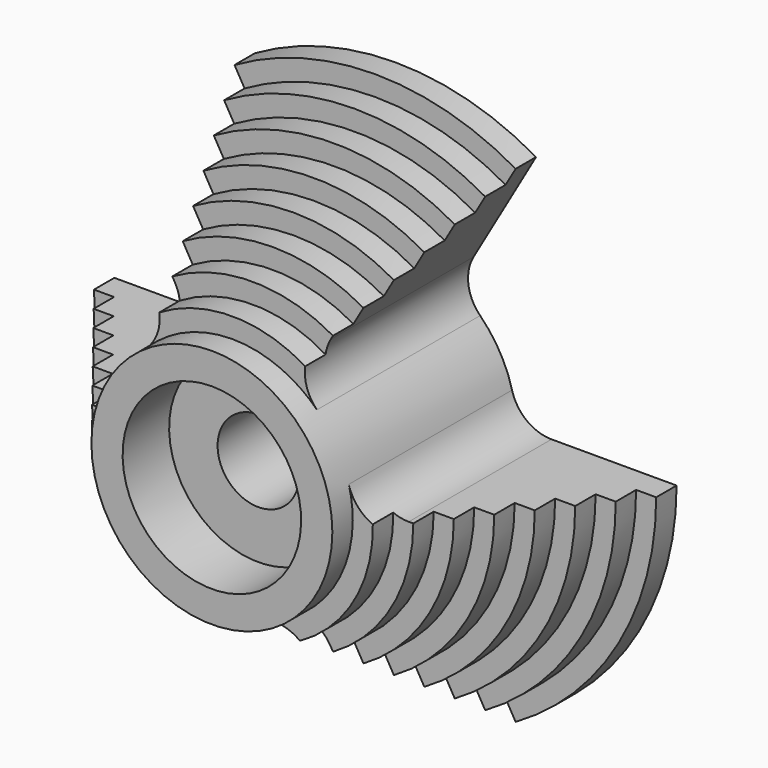
from build123d import *

# Parameters (mm, degrees)
F3_DEPTH      = 28.576
F4_T4_DEPTH   = 25.4
F4_S5_R       = 17.5
F4_T6_DEPTH   = 15
F4_T11_DEPTH  = 25.4
F4_S12_R      = 17.5
F4_T13_DEPTH  = 15
F4_T18_DEPTH  = 25.4
F4_S19_R      = 17.5
F4_T20_DEPTH  = 15
F4_T25_DEPTH  = 25.4
F4_S27_R      = 17.5
F4_T28_DEPTH  = 15
F4_T32_DEPTH  = 25.4
F4_S34_R      = 17.5
F4_T35_DEPTH  = 15
F4_T39_DEPTH  = 25.4
F4_S41_R      = 17.5
F4_T42_DEPTH  = 15
F4_T46_DEPTH  = 25.4
F4_S47_R      = 17.5
F4_T48_DEPTH  = 15
F4_T53_DEPTH  = 25.4
F4_S54_R      = 17.5
F4_T55_DEPTH  = 15
F4_T60_DEPTH  = 25.4
F4_S61_R      = 17.5
F4_T62_DEPTH  = 15
F4_T67_DEPTH  = 25.4
F4_S69_R      = 17.5
F4_T70_DEPTH  = 15
F4_T74_DEPTH  = 25.4
F4_S76_R      = 17.5
F4_T77_DEPTH  = 15
F4_T81_DEPTH  = 25.4
F4_S83_R      = 17.5
F4_T84_DEPTH  = 15
F4_T88_DEPTH  = 25.4
F4_S89_R      = 17.5
F4_T90_DEPTH  = 15
F4_T95_DEPTH  = 25.4
F4_S96_R      = 17.5
F4_T97_DEPTH  = 15
F4_T102_DEPTH = 25.4
F4_S103_R     = 17.5
F4_T104_DEPTH = 15
F4_T109_DEPTH = 25.4
F4_S111_R     = 17.5
F4_T112_DEPTH = 15
F4_T116_DEPTH = 25.4
F4_S118_R     = 17.5
F4_T119_DEPTH = 15
F4_T123_DEPTH = 25.4
F4_S125_R     = 17.5
F4_T126_DEPTH = 15


# Not quite as in the source:
# - a fillet or chamfer that OpenCascade refuses, or shapes differently, is made with other operations: its cross-section is extruded or revolved along the edge and cut away or added


with BuildPart() as f1:
    # F0 (on Right) → F1 (revolve)
    with BuildSketch(Plane.YZ):
        Polygon((0, 15), (0, 11.1125), (7.239, 11.1125), (7.239, 5.08), (21.336, 5.08), (21.336, 11.1125), (28.575, 11.1125), (28.575, 35), (25.4, 35), (25.4, 32.5), (22.225, 32.5), (22.225, 30), (19.05, 30), (19.05, 27.5), (15.875, 27.5), (15.875, 25), (12.7, 25), (12.7, 22.5), (9.525, 22.5), (9.525, 20), (6.35, 20), (6.35, 17.5), (3.175, 17.5), (3.175, 15), align=None)
    revolve(axis=Axis((0, 14.2875, 0), (0, 1, 0)))

    # F2 (on Front) → F3 (cut, through all)
    with BuildSketch(Plane.XZ):
        with BuildLine():
            ThreePointArc((-15, 0), (-12.9903810568, 7.5), (-7.5, 12.9903810568))
            Line((-7.5, 12.9903810568), (-17.5, 30.3108891325))
            ThreePointArc((-17.5, 30.3108891325), (-30.3108891325, 17.5), (-35, 0))
            Line((-35, 0), (-15, 0))
        make_face()
        with BuildLine():
            ThreePointArc((7.5, 12.9903810568), (12.9903810568, 7.5), (15, 0))
            Line((15, 0), (35, 0))
            ThreePointArc((35, 0), (30.3108891325, 17.5), (17.5, 30.3108891325))
            Line((17.5, 30.3108891325), (7.5, 12.9903810568))
        make_face()
        with BuildLine():
            Line((17.5, -30.3108891325), (7.5, -12.9903810568))
            ThreePointArc((7.5, -12.9903810568), (0, -15), (-7.5, -12.9903810568))
            Line((-7.5, -12.9903810568), (-17.5, -30.3108891325))
            ThreePointArc((-17.5, -30.3108891325), (0, -35), (17.5, -30.3108891325))
        make_face()
    extrude(amount=-F3_DEPTH, mode=Mode.SUBTRACT)

    # F4: fillet of radius 5.08 on 6 edges, made by hand


with BuildPart() as f4_tool2:
    # F4_s3 → F4_t4 (new body)
    with BuildSketch(Plane.XZ.offset(-3.175)):
        with BuildLine():
            ThreePointArc((19.4267856322, 0), (16.3221367597, 1.059110126), (14.5120410599, 3.7948207171))
            ThreePointArc((14.5120410599, 3.7948207171), (14.8775101394, 1.9130321614), (15, 0))
            Line((15, 0), (19.4267856322, 0))
        make_face()
    extrude(amount=-F4_T4_DEPTH)

    # F4_s5 → F4_t6 (intersect, symmetric)
    with BuildSketch(Plane.XZ.offset(-15.9)):
        Circle(F4_S5_R)
    extrude(amount=F4_T6_DEPTH, both=True, mode=Mode.INTERSECT)

    split(bisect_by=Plane.XZ.offset(-6.35), keep=Keep.TOP)


with BuildPart() as f1_1:
    add(f1.part)

    # F4_t1: union F4_tool2
    add(f4_tool2.part)


with BuildPart() as f4_tool9:
    # F4_s10 → F4_t11 (new body)
    with BuildSketch(Plane.XZ.offset(-3.175)):
        with BuildLine():
            ThreePointArc((19.4267856322, 0), (16.3221367597, 1.059110126), (14.5120410599, 3.7948207171))
            ThreePointArc((14.5120410599, 3.7948207171), (14.8775101394, 1.9130321614), (15, 0))
            Line((15, 0), (19.4267856322, 0))
        make_face()
    extrude(amount=-F4_T11_DEPTH)

    # F4_s12 → F4_t13 (cut, symmetric)
    with BuildSketch(Plane.XZ.offset(-15.9)):
        Circle(F4_S12_R)
    extrude(amount=F4_T13_DEPTH, both=True, mode=Mode.SUBTRACT)

    split(bisect_by=Plane.XZ.offset(-6.35), keep=Keep.BOTTOM)


with BuildPart() as f1_2:
    add(f1_1.part)

    # F4_t8: union F4_tool9
    add(f4_tool9.part)


with BuildPart() as f4_tool16:
    # F4_s17 → F4_t18 (new body)
    with BuildSketch(Plane.XZ.offset(-3.175)):
        with BuildLine():
            ThreePointArc((19.4267856322, 0), (16.3221367597, 1.059110126), (14.5120410599, 3.7948207171))
            ThreePointArc((14.5120410599, 3.7948207171), (14.8775101394, 1.9130321614), (15, 0))
            Line((15, 0), (19.4267856322, 0))
        make_face()
    extrude(amount=-F4_T18_DEPTH)

    # F4_s19 → F4_t20 (intersect, symmetric)
    with BuildSketch(Plane.XZ.offset(-15.9)):
        Circle(F4_S19_R)
    extrude(amount=F4_T20_DEPTH, both=True, mode=Mode.INTERSECT)

    split(bisect_by=Plane.XZ.offset(-6.35), keep=Keep.BOTTOM)


with BuildPart() as f1_3:
    add(f1_2.part)

    # F4_t15: union F4_tool16
    add(f4_tool16.part)


with BuildPart() as f4_tool23:
    # F4_s24 → F4_t25 (new body)
    with BuildSketch(Plane.XZ.offset(-3.175)):
        with BuildLine():
            ThreePointArc((9.7133928161, 16.8240898714), (9.0782846544, 13.6058300149), (10.5424316738, 10.6703858601))
            ThreePointArc((10.5424316738, 10.6703858601), (9.0954895198, 11.9277856451), (7.5, 12.9903810568))
            Line((7.5, 12.9903810568), (9.7133928161, 16.8240898714))
        make_face()
    extrude(amount=-F4_T25_DEPTH)

    split(bisect_by=Plane.XZ.offset(-6.35), keep=Keep.TOP)

    # F4_s27 → F4_t28 (intersect, symmetric)
    with BuildSketch(Plane.XZ.offset(-15.9)):
        Circle(F4_S27_R)
    extrude(amount=F4_T28_DEPTH, both=True, mode=Mode.INTERSECT)


with BuildPart() as f1_4:
    add(f1_3.part)

    # F4_t22: union F4_tool23
    add(f4_tool23.part)


with BuildPart() as f4_tool30:
    # F4_s31 → F4_t32 (new body)
    with BuildSketch(Plane.XZ.offset(-3.175)):
        with BuildLine():
            ThreePointArc((9.7133928161, 16.8240898714), (9.0782846544, 13.6058300149), (10.5424316738, 10.6703858601))
            ThreePointArc((10.5424316738, 10.6703858601), (9.0954895198, 11.9277856451), (7.5, 12.9903810568))
            Line((7.5, 12.9903810568), (9.7133928161, 16.8240898714))
        make_face()
    extrude(amount=-F4_T32_DEPTH)

    split(bisect_by=Plane.XZ.offset(-6.35), keep=Keep.BOTTOM)

    # F4_s34 → F4_t35 (cut, symmetric)
    with BuildSketch(Plane.XZ.offset(-15.9)):
        Circle(F4_S34_R)
    extrude(amount=F4_T35_DEPTH, both=True, mode=Mode.SUBTRACT)


with BuildPart() as f1_5:
    add(f1_4.part)

    # F4_t29: union F4_tool30
    add(f4_tool30.part)


with BuildPart() as f4_tool37:
    # F4_s38 → F4_t39 (new body)
    with BuildSketch(Plane.XZ.offset(-3.175)):
        with BuildLine():
            ThreePointArc((9.7133928161, 16.8240898714), (9.0782846544, 13.6058300149), (10.5424316738, 10.6703858601))
            ThreePointArc((10.5424316738, 10.6703858601), (9.0954895198, 11.9277856451), (7.5, 12.9903810568))
            Line((7.5, 12.9903810568), (9.7133928161, 16.8240898714))
        make_face()
    extrude(amount=-F4_T39_DEPTH)

    split(bisect_by=Plane.XZ.offset(-6.35), keep=Keep.BOTTOM)

    # F4_s41 → F4_t42 (intersect, symmetric)
    with BuildSketch(Plane.XZ.offset(-15.9)):
        Circle(F4_S41_R)
    extrude(amount=F4_T42_DEPTH, both=True, mode=Mode.INTERSECT)


with BuildPart() as f1_6:
    add(f1_5.part)

    # F4_t36: union F4_tool37
    add(f4_tool37.part)


with BuildPart() as f4_tool44:
    # F4_s45 → F4_t46 (new body)
    with BuildSketch(Plane.XZ.offset(-3.175)):
        with BuildLine():
            ThreePointArc((-10.5424316738, 10.6703858601), (-9.0782846544, 13.6058300149), (-9.7133928161, 16.8240898714))
            Line((-9.7133928161, 16.8240898714), (-7.5, 12.9903810568))
            ThreePointArc((-7.5, 12.9903810568), (-9.0954895198, 11.9277856451), (-10.5424316738, 10.6703858601))
        make_face()
    extrude(amount=-F4_T46_DEPTH)

    # F4_s47 → F4_t48 (intersect, symmetric)
    with BuildSketch(Plane.XZ.offset(-15.9)):
        Circle(F4_S47_R)
    extrude(amount=F4_T48_DEPTH, both=True, mode=Mode.INTERSECT)

    split(bisect_by=Plane.XZ.offset(-6.35), keep=Keep.TOP)


with BuildPart() as f1_7:
    add(f1_6.part)

    # F4_t43: union F4_tool44
    add(f4_tool44.part)


with BuildPart() as f4_tool51:
    # F4_s52 → F4_t53 (new body)
    with BuildSketch(Plane.XZ.offset(-3.175)):
        with BuildLine():
            ThreePointArc((-10.5424316738, 10.6703858601), (-9.0782846544, 13.6058300149), (-9.7133928161, 16.8240898714))
            Line((-9.7133928161, 16.8240898714), (-7.5, 12.9903810568))
            ThreePointArc((-7.5, 12.9903810568), (-9.0954895198, 11.9277856451), (-10.5424316738, 10.6703858601))
        make_face()
    extrude(amount=-F4_T53_DEPTH)

    # F4_s54 → F4_t55 (intersect, symmetric)
    with BuildSketch(Plane.XZ.offset(-15.9)):
        Circle(F4_S54_R)
    extrude(amount=F4_T55_DEPTH, both=True, mode=Mode.INTERSECT)

    split(bisect_by=Plane.XZ.offset(-6.35), keep=Keep.BOTTOM)


with BuildPart() as f1_8:
    add(f1_7.part)

    # F4_t50: union F4_tool51
    add(f4_tool51.part)


with BuildPart() as f4_tool58:
    # F4_s59 → F4_t60 (new body)
    with BuildSketch(Plane.XZ.offset(-3.175)):
        with BuildLine():
            ThreePointArc((-10.5424316738, 10.6703858601), (-9.0782846544, 13.6058300149), (-9.7133928161, 16.8240898714))
            Line((-9.7133928161, 16.8240898714), (-7.5, 12.9903810568))
            ThreePointArc((-7.5, 12.9903810568), (-9.0954895198, 11.9277856451), (-10.5424316738, 10.6703858601))
        make_face()
    extrude(amount=-F4_T60_DEPTH)

    # F4_s61 → F4_t62 (cut, symmetric)
    with BuildSketch(Plane.XZ.offset(-15.9)):
        Circle(F4_S61_R)
    extrude(amount=F4_T62_DEPTH, both=True, mode=Mode.SUBTRACT)

    split(bisect_by=Plane.XZ.offset(-6.35), keep=Keep.BOTTOM)


with BuildPart() as f1_9:
    add(f1_8.part)

    # F4_t57: union F4_tool58
    add(f4_tool58.part)


with BuildPart() as f4_tool65:
    # F4_s66 → F4_t67 (new body)
    with BuildSketch(Plane.XZ.offset(-3.175)):
        with BuildLine():
            ThreePointArc((-19.4267856322, 0), (-16.3221367597, 1.059110126), (-14.5120410599, 3.7948207171))
            ThreePointArc((-14.5120410599, 3.7948207171), (-14.8775101394, 1.9130321614), (-15, 0))
            Line((-15, 0), (-19.4267856322, 0))
        make_face()
    extrude(amount=-F4_T67_DEPTH)

    split(bisect_by=Plane.XZ.offset(-6.35), keep=Keep.TOP)

    # F4_s69 → F4_t70 (intersect, symmetric)
    with BuildSketch(Plane.XZ.offset(-15.9)):
        Circle(F4_S69_R)
    extrude(amount=F4_T70_DEPTH, both=True, mode=Mode.INTERSECT)


with BuildPart() as f1_10:
    add(f1_9.part)

    # F4_t64: union F4_tool65
    add(f4_tool65.part)


with BuildPart() as f4_tool72:
    # F4_s73 → F4_t74 (new body)
    with BuildSketch(Plane.XZ.offset(-3.175)):
        with BuildLine():
            ThreePointArc((-19.4267856322, 0), (-16.3221367597, 1.059110126), (-14.5120410599, 3.7948207171))
            ThreePointArc((-14.5120410599, 3.7948207171), (-14.8775101394, 1.9130321614), (-15, 0))
            Line((-15, 0), (-19.4267856322, 0))
        make_face()
    extrude(amount=-F4_T74_DEPTH)

    split(bisect_by=Plane.XZ.offset(-6.35), keep=Keep.BOTTOM)

    # F4_s76 → F4_t77 (cut, symmetric)
    with BuildSketch(Plane.XZ.offset(-15.9)):
        Circle(F4_S76_R)
    extrude(amount=F4_T77_DEPTH, both=True, mode=Mode.SUBTRACT)


with BuildPart() as f1_11:
    add(f1_10.part)

    # F4_t71: union F4_tool72
    add(f4_tool72.part)


with BuildPart() as f4_tool79:
    # F4_s80 → F4_t81 (new body)
    with BuildSketch(Plane.XZ.offset(-3.175)):
        with BuildLine():
            ThreePointArc((-19.4267856322, 0), (-16.3221367597, 1.059110126), (-14.5120410599, 3.7948207171))
            ThreePointArc((-14.5120410599, 3.7948207171), (-14.8775101394, 1.9130321614), (-15, 0))
            Line((-15, 0), (-19.4267856322, 0))
        make_face()
    extrude(amount=-F4_T81_DEPTH)

    split(bisect_by=Plane.XZ.offset(-6.35), keep=Keep.BOTTOM)

    # F4_s83 → F4_t84 (intersect, symmetric)
    with BuildSketch(Plane.XZ.offset(-15.9)):
        Circle(F4_S83_R)
    extrude(amount=F4_T84_DEPTH, both=True, mode=Mode.INTERSECT)


with BuildPart() as f1_12:
    add(f1_11.part)

    # F4_t78: union F4_tool79
    add(f4_tool79.part)


with BuildPart() as f4_tool86:
    # F4_s87 → F4_t88 (new body)
    with BuildSketch(Plane.XZ.offset(-3.175)):
        with BuildLine():
            ThreePointArc((-9.7133928161, -16.8240898714), (-7.2438521053, -14.664940141), (-3.9696093861, -14.4652065772))
            ThreePointArc((-3.9696093861, -14.4652065772), (-5.7820206197, -13.8408178065), (-7.5, -12.9903810568))
            Line((-7.5, -12.9903810568), (-9.7133928161, -16.8240898714))
        make_face()
    extrude(amount=-F4_T88_DEPTH)

    # F4_s89 → F4_t90 (intersect, symmetric)
    with BuildSketch(Plane.XZ.offset(-15.9)):
        Circle(F4_S89_R)
    extrude(amount=F4_T90_DEPTH, both=True, mode=Mode.INTERSECT)

    split(bisect_by=Plane.XZ.offset(-6.35), keep=Keep.TOP)


with BuildPart() as f1_13:
    add(f1_12.part)

    # F4_t85: union F4_tool86
    add(f4_tool86.part)


with BuildPart() as f4_tool93:
    # F4_s94 → F4_t95 (new body)
    with BuildSketch(Plane.XZ.offset(-3.175)):
        with BuildLine():
            ThreePointArc((-9.7133928161, -16.8240898714), (-7.2438521053, -14.664940141), (-3.9696093861, -14.4652065772))
            ThreePointArc((-3.9696093861, -14.4652065772), (-5.7820206197, -13.8408178065), (-7.5, -12.9903810568))
            Line((-7.5, -12.9903810568), (-9.7133928161, -16.8240898714))
        make_face()
    extrude(amount=-F4_T95_DEPTH)

    # F4_s96 → F4_t97 (cut, symmetric)
    with BuildSketch(Plane.XZ.offset(-15.9)):
        Circle(F4_S96_R)
    extrude(amount=F4_T97_DEPTH, both=True, mode=Mode.SUBTRACT)

    split(bisect_by=Plane.XZ.offset(-6.35), keep=Keep.BOTTOM)


with BuildPart() as f1_14:
    add(f1_13.part)

    # F4_t92: union F4_tool93
    add(f4_tool93.part)


with BuildPart() as f4_tool100:
    # F4_s101 → F4_t102 (new body)
    with BuildSketch(Plane.XZ.offset(-3.175)):
        with BuildLine():
            ThreePointArc((-9.7133928161, -16.8240898714), (-7.2438521053, -14.664940141), (-3.9696093861, -14.4652065772))
            ThreePointArc((-3.9696093861, -14.4652065772), (-5.7820206197, -13.8408178065), (-7.5, -12.9903810568))
            Line((-7.5, -12.9903810568), (-9.7133928161, -16.8240898714))
        make_face()
    extrude(amount=-F4_T102_DEPTH)

    # F4_s103 → F4_t104 (intersect, symmetric)
    with BuildSketch(Plane.XZ.offset(-15.9)):
        Circle(F4_S103_R)
    extrude(amount=F4_T104_DEPTH, both=True, mode=Mode.INTERSECT)

    split(bisect_by=Plane.XZ.offset(-6.35), keep=Keep.BOTTOM)


with BuildPart() as f1_15:
    add(f1_14.part)

    # F4_t99: union F4_tool100
    add(f4_tool100.part)


with BuildPart() as f4_tool107:
    # F4_s108 → F4_t109 (new body)
    with BuildSketch(Plane.XZ.offset(-3.175)):
        with BuildLine():
            ThreePointArc((9.7133928161, -16.8240898714), (7.2438521053, -14.664940141), (3.9696093861, -14.4652065772))
            ThreePointArc((3.9696093861, -14.4652065772), (5.7820206197, -13.8408178065), (7.5, -12.9903810568))
            Line((7.5, -12.9903810568), (9.7133928161, -16.8240898714))
        make_face()
    extrude(amount=-F4_T109_DEPTH)

    split(bisect_by=Plane.XZ.offset(-6.35), keep=Keep.TOP)

    # F4_s111 → F4_t112 (intersect, symmetric)
    with BuildSketch(Plane.XZ.offset(-15.9)):
        Circle(F4_S111_R)
    extrude(amount=F4_T112_DEPTH, both=True, mode=Mode.INTERSECT)


with BuildPart() as f1_16:
    add(f1_15.part)

    # F4_t106: union F4_tool107
    add(f4_tool107.part)


with BuildPart() as f4_tool114:
    # F4_s115 → F4_t116 (new body)
    with BuildSketch(Plane.XZ.offset(-3.175)):
        with BuildLine():
            ThreePointArc((9.7133928161, -16.8240898714), (7.2438521053, -14.664940141), (3.9696093861, -14.4652065772))
            ThreePointArc((3.9696093861, -14.4652065772), (5.7820206197, -13.8408178065), (7.5, -12.9903810568))
            Line((7.5, -12.9903810568), (9.7133928161, -16.8240898714))
        make_face()
    extrude(amount=-F4_T116_DEPTH)

    split(bisect_by=Plane.XZ.offset(-6.35), keep=Keep.BOTTOM)

    # F4_s118 → F4_t119 (cut, symmetric)
    with BuildSketch(Plane.XZ.offset(-15.9)):
        Circle(F4_S118_R)
    extrude(amount=F4_T119_DEPTH, both=True, mode=Mode.SUBTRACT)


with BuildPart() as f1_17:
    add(f1_16.part)

    # F4_t113: union F4_tool114
    add(f4_tool114.part)


with BuildPart() as f4_tool121:
    # F4_s122 → F4_t123 (new body)
    with BuildSketch(Plane.XZ.offset(-3.175)):
        with BuildLine():
            ThreePointArc((9.7133928161, -16.8240898714), (7.2438521053, -14.664940141), (3.9696093861, -14.4652065772))
            ThreePointArc((3.9696093861, -14.4652065772), (5.7820206197, -13.8408178065), (7.5, -12.9903810568))
            Line((7.5, -12.9903810568), (9.7133928161, -16.8240898714))
        make_face()
    extrude(amount=-F4_T123_DEPTH)

    split(bisect_by=Plane.XZ.offset(-6.35), keep=Keep.BOTTOM)

    # F4_s125 → F4_t126 (intersect, symmetric)
    with BuildSketch(Plane.XZ.offset(-15.9)):
        Circle(F4_S125_R)
    extrude(amount=F4_T126_DEPTH, both=True, mode=Mode.INTERSECT)


with BuildPart() as f1_18:
    add(f1_17.part)

    # F4_t120: union F4_tool121
    add(f4_tool121.part)


solid = f1_18.part
